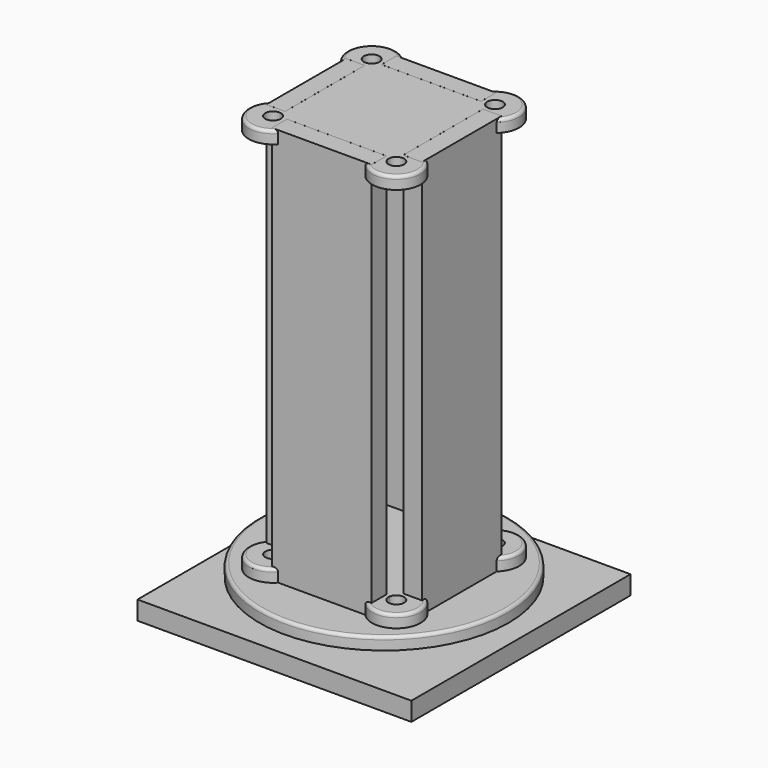
from build123d import *

# Parameters (mm, degrees)
F0_W      = 279.4
F0_H      = 279.4
F1_DEPTH  = 19.05
F2_W      = 152.4
F2_H      = 152.4
F3_DEPTH  = 8.89
F5_R      = 127
F6_DEPTH  = 12.7
F7_W      = 101.6
F7_H      = 19.05
F7_W_2    = 19.05
F7_H_2    = 101.6
F8_DEPTH  = 406.4
F21_DEPTH = 12.7
F22_R     = 3.175
F24_R     = 7.9375
F25_DEPTH = 12.7
F26_R     = 3.175
F27_R     = 3.175


# Not quite as in the source:
# - the program builds the solid bodies; features that only make, move or delete a surface that nothing else refers to are left out


with BuildPart() as f1:
    # F0 (on Top) → F1 (new body)
    with BuildSketch(Plane.XY):
        Rectangle(F0_W, F0_H)
    extrude(amount=F1_DEPTH)

    # F2 (on face) → F3 (join)
    with BuildSketch(Plane.XY.offset(19.05)):
        Rectangle(F2_W, F2_H)
    extrude(amount=F3_DEPTH)

    # F5 (on offset) → F6 (join)
    with BuildSketch(Plane.XY.offset(27.94)):
        Circle(F5_R)
    extrude(amount=F6_DEPTH)

    # F7 (on face) → F8 (join)
    with BuildSketch(Plane.XY.offset(40.64)):
        with Locations((0, -69.85)):
            Rectangle(F7_W, F7_H)
        with Locations((-69.85, 0)):
            Rectangle(F7_W_2, F7_H_2)
        with Locations((0, 69.85)):
            Rectangle(F7_W, F7_H)
        with Locations((69.85, 0)):
            Rectangle(F7_W_2, F7_H_2)
    extrude(amount=F8_DEPTH)

    # F20 (on face) → F21 (join)
    with BuildSketch(Plane.XY.offset(40.64)):
        with BuildLine():
            Line((-50.8, -60.325), (0, -60.325))
            Line((0, -60.325), (50.8, -60.325))
            Line((50.8, -60.325), (50.8, -79.375))
            Line((50.8, -79.375), (44.45, -79.375))
            ThreePointArc((44.45, -79.375), (80.3474934763, -80.3474934763), (79.375, -44.45))
            Line((79.375, -44.45), (79.375, -50.8))
            Line((79.375, -50.8), (60.325, -50.8))
            Line((60.325, -50.8), (60.325, 0))
            Line((60.325, 0), (60.325, 50.8))
            Line((60.325, 50.8), (79.375, 50.8))
            Line((79.375, 50.8), (79.375, 44.45))
            ThreePointArc((79.375, 44.45), (80.3474934763, 80.3474934763), (44.45, 79.375))
            Line((44.45, 79.375), (50.8, 79.375))
            Line((50.8, 79.375), (50.8, 60.325))
            Line((50.8, 60.325), (0, 60.325))
            Line((0, 60.325), (-50.8, 60.325))
            Line((-50.8, 60.325), (-50.8, 79.375))
            Line((-50.8, 79.375), (-44.45, 79.375))
            ThreePointArc((-44.45, 79.375), (-80.3474934763, 80.3474934763), (-79.375, 44.45))
            Line((-79.375, 44.45), (-79.375, 50.8))
            Line((-79.375, 50.8), (-60.325, 50.8))
            Line((-60.325, 50.8), (-60.325, 0))
            Line((-60.325, 0), (-60.325, -50.8))
            Line((-60.325, -50.8), (-79.375, -50.8))
            Line((-79.375, -50.8), (-79.375, -44.45))
            ThreePointArc((-79.375, -44.45), (-80.3474934763, -80.3474934763), (-44.45, -79.375))
            Line((-44.45, -79.375), (-50.8, -79.375))
            Line((-50.8, -79.375), (-50.8, -60.325))
        make_face()
        with BuildLine():
            ThreePointArc((-61.8092019554, -54.9916168178), (-56.8869311974, -57.6311301033), (-54.9218427062, -62.8593427062))
            ThreePointArc((-54.9218427062, -62.8593427062), (-57.6332777778, -68.8336335942), (-63.9151407508, -70.7263114196))
            ThreePointArc((-63.9151407508, -70.7263114196), (-70.7323478094, -61.8056160656), (-61.8092019554, -54.9916168178))
        make_face(mode=Mode.SUBTRACT)
        with BuildLine():
            ThreePointArc((54.9916168179, -61.8092019554), (63.3855707991, -54.9393054434), (70.7968427062, -62.8593427062))
            ThreePointArc((70.7968427062, -62.8593427062), (70.7791902556, -63.3884183561), (70.7263114196, -63.9151407508))
            ThreePointArc((70.7263114196, -63.9151407508), (61.8056160655, -70.7323478094), (54.9916168179, -61.8092019554))
        make_face(mode=Mode.SUBTRACT)
        with BuildLine():
            ThreePointArc((-54.9916168179, 61.8092019554), (-63.912312172, 54.9919948968), (-70.7263114196, 63.9151407508))
            ThreePointArc((-70.7263114196, 63.9151407508), (-62.3323574384, 70.7850372628), (-54.9210855313, 62.865))
            ThreePointArc((-54.9210855313, 62.865), (-54.9387379819, 62.3359243501), (-54.9916168179, 61.8092019554))
        make_face(mode=Mode.SUBTRACT)
        with BuildLine():
            ThreePointArc((61.8092019553, 54.9916168179), (54.9919948968, 63.912312172), (63.9151407508, 70.7263114196))
            ThreePointArc((63.9151407508, 70.7263114196), (68.8374115088, 68.0867981341), (70.8025, 62.8585855313))
            ThreePointArc((70.8025, 62.8585855313), (68.0910649283, 56.8842946433), (61.8092019553, 54.9916168179))
        make_face(mode=Mode.SUBTRACT)
    extrude(amount=F21_DEPTH)

    # F22
    f22_edges = [f1.edges().sort_by_distance(p)[0] for p in [
        (-80.347493, -80.347493, 53.34),
        (80.347493, -80.347493, 53.34),
        (80.347493, 80.347493, 53.34),
        (-80.347493, 80.347493, 53.34),
    ]]
    fillet(f22_edges, radius=F22_R)

    # F27
    f27_edges = [f1.edges().sort_by_distance(p)[0] for p in [
        (-127, 0, 40.64),
    ]]
    fillet(f27_edges, radius=F27_R)


with BuildPart() as f25:
    # F24 (on offset) → F25 (new body)
    with BuildSketch(Plane.XY.offset(447.04)):
        with BuildLine():
            Line((60.2996, -0.0135466667), (60.2996, 0))
            Line((60.2996, 0), (60.2996, 50.8118533333))
            Line((60.2996, 50.8118533333), (79.4004, 50.8118533333))
            Line((79.4004, 50.8118533333), (79.4004, 44.4618533333))
            ThreePointArc((79.4004, 44.4618533333), (80.3728934763, 80.3593468097), (44.4754, 79.3868533333))
            Line((44.4754, 79.3868533333), (50.8254, 79.3868533333))
            Line((50.8254, 79.3868533333), (50.8254, 60.2860533333))
            Line((50.8254, 60.2860533333), (0.0135466667, 60.2860533333))
            Line((0.0135466667, 60.2860533333), (0, 60.2860533333))
            Line((0, 60.2860533333), (-50.8118533333, 60.2860533333))
            Line((-50.8118533333, 60.2860533333), (-50.8118533333, 79.3868533333))
            Line((-50.8118533333, 79.3868533333), (-44.4618533333, 79.3868533333))
            ThreePointArc((-44.4618533333, 79.3868533333), (-80.3593468097, 80.3593468097), (-79.3868533333, 44.4618533333))
            Line((-79.3868533333, 44.4618533333), (-79.3868533333, 50.8118533333))
            Line((-79.3868533333, 50.8118533333), (-60.2860533333, 50.8118533333))
            Line((-60.2860533333, 50.8118533333), (-60.2860533333, 0))
            Line((-60.2860533333, 0), (-60.2860533333, -0.0135466667))
            Line((-60.2860533333, -0.0135466667), (-60.2860533333, -50.8254))
            Line((-60.2860533333, -50.8254), (-79.3868533333, -50.8254))
            Line((-79.3868533333, -50.8254), (-79.3868533333, -44.4754))
            ThreePointArc((-79.3868533333, -44.4754), (-80.3593468097, -80.3728934763), (-44.4618533333, -79.4004))
            Line((-44.4618533333, -79.4004), (-50.8118533333, -79.4004))
            Line((-50.8118533333, -79.4004), (-50.8118533333, -60.2996))
            Line((-50.8118533333, -60.2996), (0, -60.2996))
            Line((0, -60.2996), (0.0135466667, -60.2996))
            Line((0.0135466667, -60.2996), (50.8254, -60.2996))
            Line((50.8254, -60.2996), (50.8254, -79.4004))
            Line((50.8254, -79.4004), (44.4754, -79.4004))
            ThreePointArc((44.4754, -79.4004), (80.3728934763, -80.3728934763), (79.4004, -44.4754))
            Line((79.4004, -44.4754), (79.4004, -50.8254))
            Line((79.4004, -50.8254), (60.2996, -50.8254))
            Line((60.2996, -50.8254), (60.2996, -0.0135466667))
        make_face()
        with Locations((-62.8711960395, -62.8847427062)):
            Circle(F24_R, mode=Mode.SUBTRACT)
        with Locations((62.8847427062, -62.8847427062)):
            Circle(F24_R, mode=Mode.SUBTRACT)
        with Locations((-62.8711960395, 62.8711960395)):
            Circle(F24_R, mode=Mode.SUBTRACT)
        with Locations((62.8847427062, 62.8711960395)):
            Circle(F24_R, mode=Mode.SUBTRACT)
    extrude(amount=-F25_DEPTH)

    # F26
    f26_edges = [f25.edges().sort_by_distance(p)[0] for p in [
        (-80.359347, -80.372893, 447.04),
        (80.372893, -80.372893, 447.04),
        (80.372893, 80.359347, 447.04),
        (-80.359347, 80.359347, 447.04),
    ]]
    fillet(f26_edges, radius=F26_R)


solid = Compound([f1.part, f25.part])
